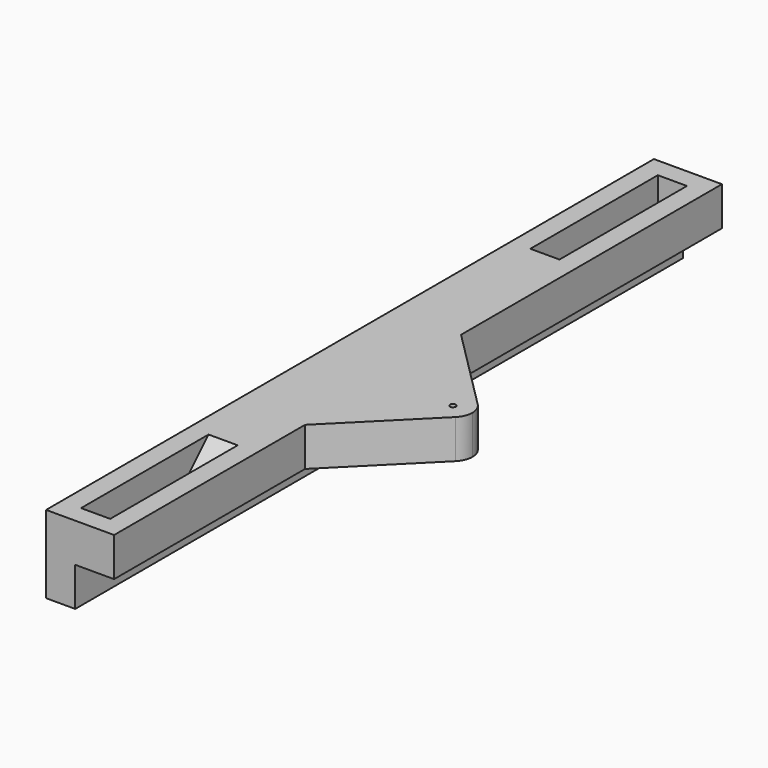
from build123d import *

# Parameters (mm, degrees)
F0_W     = 7.5
F0_H     = 41
F1_DEPTH = 20
F2_DEPTH = 10
F3_SIZE  = 9.99999
F4_W     = 10
F4_H     = 10
F5_DEPTH = 195.501
F7_DEPTH = 10
F8_R     = 0.75
F9_DEPTH = 25


# Not quite as in the source:
# - a fillet or chamfer is up to 0.001 mm smaller than in the source, because OpenCascade refuses the exact size


with BuildPart() as f1:
    # F0 (on Top) → F1 (new body)
    with BuildSketch(Plane.XY):
        Polygon((-12.5, 80), (-12.5, 75), (-12.5, -115.5), (5, -115.5), (5, -110.5), (5, 80), align=None)
        Polygon((0, 34), (0, 0), (0, -7.5), (0, -69.5), (0, -110.5), (-7.5, -110.5), (-7.5, -69.5), (-7.5, 34), (-7.5, 75), (0, 75), align=None, mode=Mode.SUBTRACT)
        with Locations((-3.75, -90)):
            Rectangle(F0_W, F0_H)
        Polygon((0, -7.5), (0, 0), (0, 34), (-7.5, 34), (-7.5, -69.5), (0, -69.5), align=None)
        with Locations((-3.75, 54.5)):
            Rectangle(F0_W, F0_H)
    extrude(amount=-F1_DEPTH)

    # F0 (on Top) → F2 (cut)
    with BuildSketch(Plane.XY):
        with Locations((-3.75, 54.5)):
            Rectangle(F0_W, F0_H)
        with Locations((-3.75, -90)):
            Rectangle(F0_W, F0_H)
    extrude(amount=-F2_DEPTH, mode=Mode.SUBTRACT)

    # F3 (size 10 in the source; OpenCascade refuses exactly that, so slightly less here)
    f3_edges = [f1.edges().sort_by_distance(p)[0] for p in [
        (-3.75, -69.5, -10),
        (-3.75, 34, -10),
    ]]
    chamfer(f3_edges, length=F3_SIZE)

    # F4 (on face) → F5 (cut, through all)
    with BuildSketch(Plane.XZ.offset(115.5)):
        with Locations((0, -15)):
            Rectangle(F4_W, F4_H)
    extrude(amount=-F5_DEPTH, mode=Mode.SUBTRACT)

    # F6 (on face) → F7 (join)
    with BuildSketch(Plane.XY):
        with BuildLine():
            Line((29, -22.6551367564), (5, -3.9060580615))
            Line((5, -3.9060580615), (5, -54.0939419385))
            Line((5, -54.0939419385), (32.0781262822, -32.9401952478))
            ThreePointArc((32.0781262822, -32.9401952478), (26.8080409916, -33.4939198597), (24, -29))
            ThreePointArc((24, -29), (25.4644660941, -25.4644660941), (29, -24))
            Line((29, -24), (29, -22.6551367564))
        make_face()
        with BuildLine():
            Line((32.0781262822, -25.0598047522), (29, -22.6551367564))
            Line((29, -22.6551367564), (29, -24))
            ThreePointArc((29, -24), (30.627732128, -24.2723697142), (32.0781262822, -25.0598047522))
        make_face()
        with BuildLine():
            ThreePointArc((32.0781262822, -25.0598047522), (30.627732128, -24.2723697142), (29, -24))
            Line((29, -24), (29, -28.5))
            ThreePointArc((29, -28.5), (29.3535533906, -28.6464466094), (29.5, -29))
            ThreePointArc((29.5, -29), (29, -29.5), (28.5, -29))
            Line((28.5, -29), (24, -29))
            ThreePointArc((24, -29), (26.8080409916, -33.4939198597), (32.0781262822, -32.9401952478))
            ThreePointArc((32.0781262822, -32.9401952478), (33.4939198597, -31.1919590084), (34, -29))
            ThreePointArc((34, -29), (33.4939198597, -26.8080409916), (32.0781262822, -25.0598047522))
        make_face()
        with BuildLine():
            Line((29, -28.5), (29, -24))
            ThreePointArc((29, -24), (25.4644660941, -25.4644660941), (24, -29))
            Line((24, -29), (28.5, -29))
            ThreePointArc((28.5, -29), (28.6464466094, -28.6464466094), (29, -28.5))
        make_face()
    extrude(amount=-F7_DEPTH)

    # F8 (on face) → F9 (cut)
    with BuildSketch(Plane(origin=(0, 0, -10), x_dir=(1, 0, 0), z_dir=(0, 0, -1))):
        with Locations((23, 29)):
            Circle(F8_R)
        with BuildLine():
            ThreePointArc((26.537409976, 32.5336568398), (27.6199052956, 30.9121911672), (28, 29))
            ThreePointArc((28, 29), (27.6199052956, 27.0878088328), (26.537409976, 25.4663431602))
            Line((26.537409976, 25.4663431602), (5, 3.9060580615))
            Line((5, 3.9060580615), (32.0781262822, 25.0598047522))
            ThreePointArc((32.0781262822, 25.0598047522), (34, 29), (32.0781262822, 32.9401952478))
            Line((32.0781262822, 32.9401952478), (5, 54.0939419385))
            Line((5, 54.0939419385), (26.537409976, 32.5336568398))
        make_face()
        with BuildLine():
            ThreePointArc((29.5, 29), (29, 28.5), (28.5, 29))
            ThreePointArc((28.5, 29), (29, 29.5), (29.5, 29))
        make_face(mode=Mode.SUBTRACT)
    extrude(amount=-F9_DEPTH, mode=Mode.SUBTRACT)


solid = f1.part
